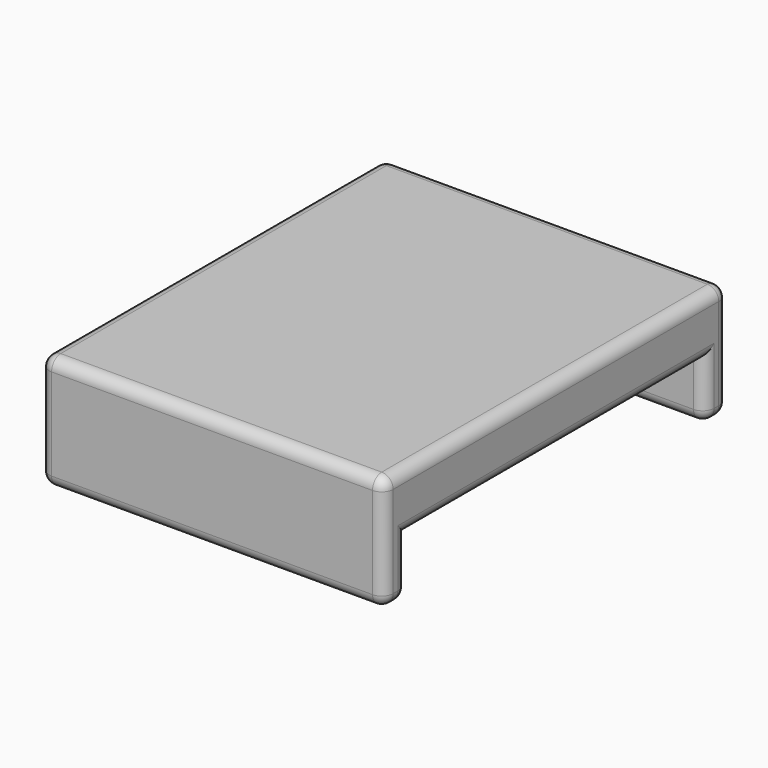
from build123d import *

# Parameters (mm, degrees)
F0_W     = 25
F0_H     = 32.5
F0_W_2   = 2.5
F1_DEPTH = 5
F2_DEPTH = 5
F3_R     = 1


with BuildPart() as f1:
    # F0 (on Top) → F1 (new body)
    with BuildSketch(Plane.XY):
        Rectangle(F0_W, F0_H)
        Polygon((-15, 16.25), (-12.5, 16.25), (12.5, 16.25), (15, 16.25), (15, 18.75), (-15, 18.75), align=None)
        with Locations((-13.75, 0)):
            Rectangle(F0_W_2, F0_H)
        Polygon((12.5, -16.25), (-12.5, -16.25), (-15, -16.25), (-15, -18.75), (15, -18.75), (15, -16.25), align=None)
        with Locations((13.75, 0)):
            Rectangle(F0_W_2, F0_H)
    extrude(amount=F1_DEPTH)

    # F0 (on Top) → F2 (join)
    with BuildSketch(Plane.XY):
        Polygon((12.5, -16.25), (-12.5, -16.25), (-15, -16.25), (-15, -18.75), (15, -18.75), (15, -16.25), align=None)
        Polygon((-15, 16.25), (-12.5, 16.25), (12.5, 16.25), (15, 16.25), (15, 18.75), (-15, 18.75), align=None)
    extrude(amount=-F2_DEPTH)

    # F3
    f3_edges = [f1.edges().sort_by_distance(p)[0] for p in [
        (0, 16.25, -5),
        (15, 17.5, -5),
        (0, 18.75, -5),
        (-15, 17.5, -5),
        (-15, -17.5, -5),
        (0, -18.75, -5),
        (15, -17.5, -5),
        (0, -16.25, -5),
        (-15, 0, 5),
        (-15, -18.75, 0),
        (-15, -16.25, -2.5),
        (-15, 0, 0),
        (-15, 16.25, -2.5),
        (-15, 18.75, 0),
        (15, 18.75, 0),
        (0, 18.75, 5),
        (15, -18.75, 0),
        (15, 0, 5),
        (15, 16.25, -2.5),
        (15, 0, 0),
        (15, -16.25, -2.5),
        (0, -18.75, 5),
    ]]
    fillet(f3_edges, radius=F3_R)


solid = f1.part
